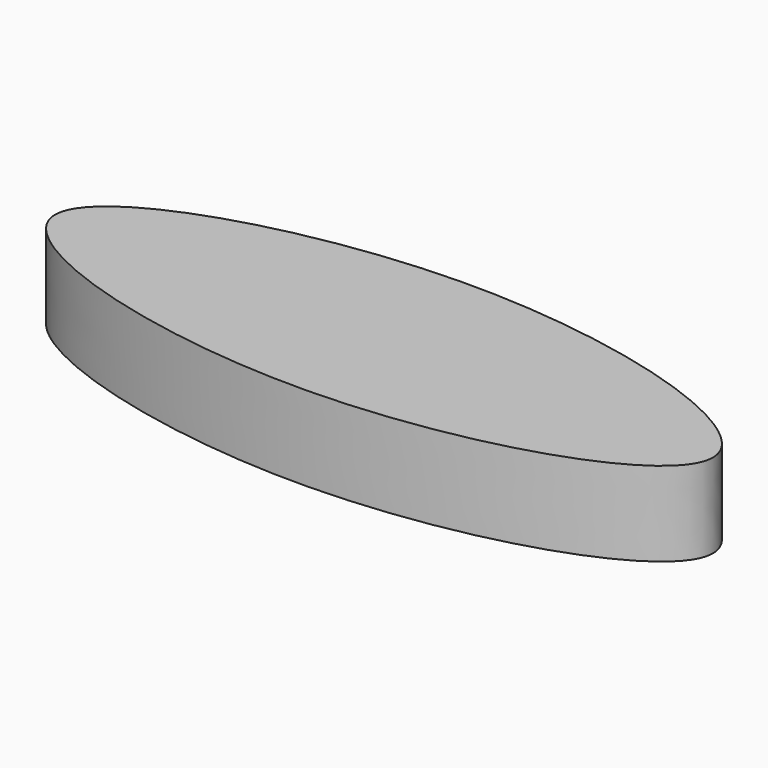
from build123d import *

# Parameters (mm, degrees)
F1_DEPTH  = 5
F2_SCALE  = 1.25
F11_R     = 3.625
F13_DEPTH = 3.25
F15_R     = 4.297586673
F16_DEPTH = 1.2


# Not quite as in the source:
# - a feature of the source that left no trace in its solid (it failed there, or was rolled back) is left out


with BuildPart() as f1:
    # F0 (on Top) → F1 (new body)
    with BuildSketch(Plane.XY):
        with BuildLine():
            Line((-19.5, 0), (0, 0))
            Line((0, 0), (0, 6.5))
            add(Edge.make_bspline(
                [(-19.5, 0), (-19.5, 3.25), (-9.75, 6.5), (0, 6.5)],
                knots=[0, 0, 0, 0, 0.25, 0.25, 0.25, 0.25], degree=3))
        make_face()
        with BuildLine():
            Line((0, 6.5), (0, 0))
            Line((0, 0), (19.5, 0))
            add(Edge.make_bspline(
                [(0, 6.5), (9.75, 6.5), (19.5, 3.25), (19.5, 0)],
                knots=[0.25, 0.25, 0.25, 0.25, 0.5, 0.5, 0.5, 0.5], degree=3))
        make_face()
        with BuildLine():
            Line((19.5, 0), (0, 0))
            Line((0, 0), (0, -6.5))
            add(Edge.make_bspline(
                [(19.5, 0), (19.5, -3.25), (9.75, -6.5), (0, -6.5)],
                knots=[0.5, 0.5, 0.5, 0.5, 0.75, 0.75, 0.75, 0.75], degree=3))
        make_face()
        with BuildLine():
            Line((0, -6.5), (0, 0))
            Line((0, 0), (-19.5, 0))
            add(Edge.make_bspline(
                [(0, -6.5), (-9.75, -6.5), (-19.5, -3.25), (-19.5, 0)],
                knots=[0.75, 0.75, 0.75, 0.75, 1, 1, 1, 1], degree=3))
        make_face()
    extrude(amount=F1_DEPTH)


with BuildPart() as f2_1:
    # F2: copy of F1
    add(f1.part.scale(F2_SCALE))

    # F5: cut F1
    add(f1.part, mode=Mode.SUBTRACT)

    # F11 (on face) → F13 (cut)
    with BuildSketch(Plane(origin=(0, 0, 5), x_dir=(1, 0, 0), z_dir=(0, 0, -1))):
        Circle(F11_R)
    extrude(amount=-F13_DEPTH, mode=Mode.SUBTRACT)


with BuildPart() as f14_1:
    # F14: copy of F2_1
    add(f2_1.part.moved(Location((-4.8109386116, 41.9865772128, 0))))

    # F15 (on face) → F16 (join)
    with BuildSketch(Plane.XY.offset(6.25)):
        with Locations((-4.8109386116, 41.9865772128)):
            Circle(F15_R)
    extrude(amount=-F16_DEPTH)


with BuildPart() as f17_1:
    # F17: copy of F14_1
    add(f14_1.part)


solid = f14_1.part
